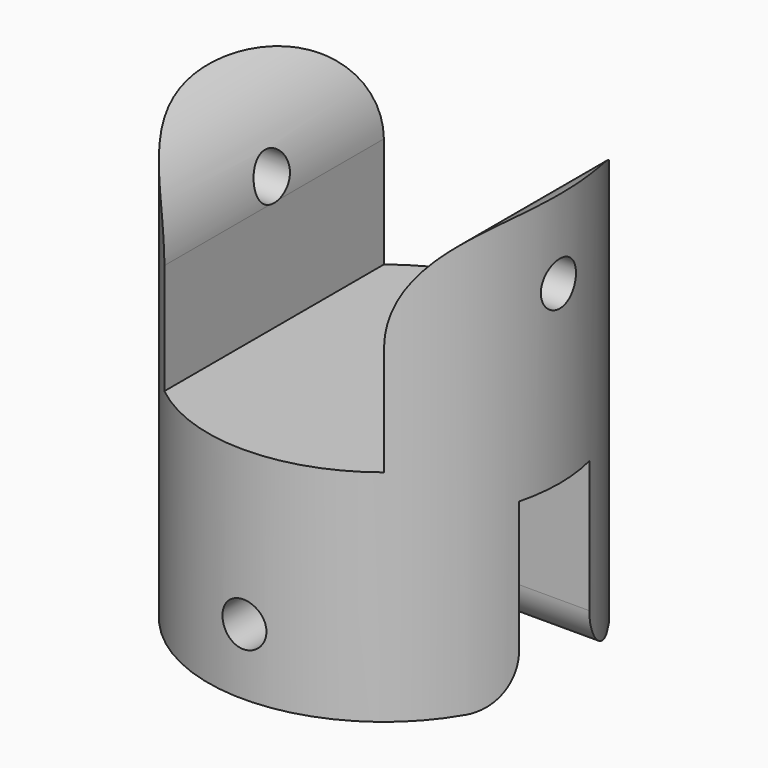
from build123d import *

# Parameters (mm, degrees)
F0_R         = 8
F1_DEPTH     = 20
F2_W         = 10
F2_H         = 24
F3_DEPTH     = 10
F4_W         = 19
F4_H         = 4
F5_DEPTH     = 8
F6_R         = 1
F7_DEPTH     = 5
F8_R         = 1
F9_DEPTH     = 5
F10_R        = 1
F11_DEPTH    = 8
F12_T1_DEPTH = 37.4894960018
F13_R        = 2


# Not quite as in the source:
# - a fillet or chamfer that OpenCascade refuses, or shapes differently, is made with other operations: its cross-section is extruded or revolved along the edge and cut away or added


with BuildPart() as f1:
    # F0 (on Top) → F1 (new body)
    with BuildSketch(Plane.XY):
        Circle(F0_R)
    extrude(amount=F1_DEPTH)

    # F2 (on face) → F3 (cut)
    with BuildSketch(Plane.XY.offset(20)):
        Rectangle(F2_W, F2_H)
    extrude(amount=-F3_DEPTH, mode=Mode.SUBTRACT)

    # F4 (on face) → F5 (cut)
    with BuildSketch(Plane(origin=(0, 0, 0), x_dir=(1, 0, 0), z_dir=(0, 0, -1))):
        Rectangle(F4_W, F4_H)
    extrude(amount=-F5_DEPTH, mode=Mode.SUBTRACT)

    # F6 (on face) → F7 (cut)
    with BuildSketch(Plane.YZ.offset(-5)):
        with Locations((1.8555e-06, 16)):
            Circle(F6_R)
    extrude(amount=-F7_DEPTH, mode=Mode.SUBTRACT)

    # F8 (on face) → F9 (cut)
    with BuildSketch(Plane(origin=(5, 0, 0), x_dir=(0, -1, 0), z_dir=(-1, 0, 0))):
        with Locations((0, 16)):
            Circle(F8_R)
    extrude(amount=-F9_DEPTH, mode=Mode.SUBTRACT)

    # F10 (on Front) → F11 (cut, symmetric)
    with BuildSketch(Plane.XZ):
        with Locations((0, 3)):
            Circle(F10_R)
    extrude(amount=F11_DEPTH, both=True, mode=Mode.SUBTRACT)

    # F12: fillet of radius 5 on 2 edges, made by hand

    # F12_s2 → F12_t1 (cut)
    with BuildSketch(Plane.XZ.offset(-18.7447480009)):
        with BuildLine():
            ThreePointArc((-9.9999, 20.0001), (-6.4643660941, 18.5356339059), (-4.9999, 15.0001))
            Line((-4.9999, 15.0001), (-4.8999, 15.0001))
            ThreePointArc((-4.8999, 15.0001), (-4.9, 17.50005), (-4.9, 20))
            Line((-4.9, 20), (-5, 20.1))
            ThreePointArc((-5, 20.1), (-7.49995, 20.1), (-9.9999, 20.1001))
            Line((-9.9999, 20.1001), (-9.9999, 20.0001))
        make_face()
        with BuildLine():
            ThreePointArc((4.9999, 15.0001), (6.4643660941, 18.5356339059), (9.9999, 20.0001))
            Line((9.9999, 20.0001), (9.9999, 20.1001))
            ThreePointArc((9.9999, 20.1001), (7.49995, 20.1), (5, 20.1))
            Line((5, 20.1), (4.9, 20))
            ThreePointArc((4.9, 20), (4.9, 17.50005), (4.8999, 15.0001))
            Line((4.8999, 15.0001), (4.9999, 15.0001))
        make_face()
    extrude(amount=F12_T1_DEPTH, mode=Mode.SUBTRACT)

    # F13
    f13_edges = [f1.edges().sort_by_distance(p)[0] for p in [
        (0, -2, 0),
        (0, 2, 0),
    ]]
    fillet(f13_edges, radius=F13_R)


solid = f1.part
